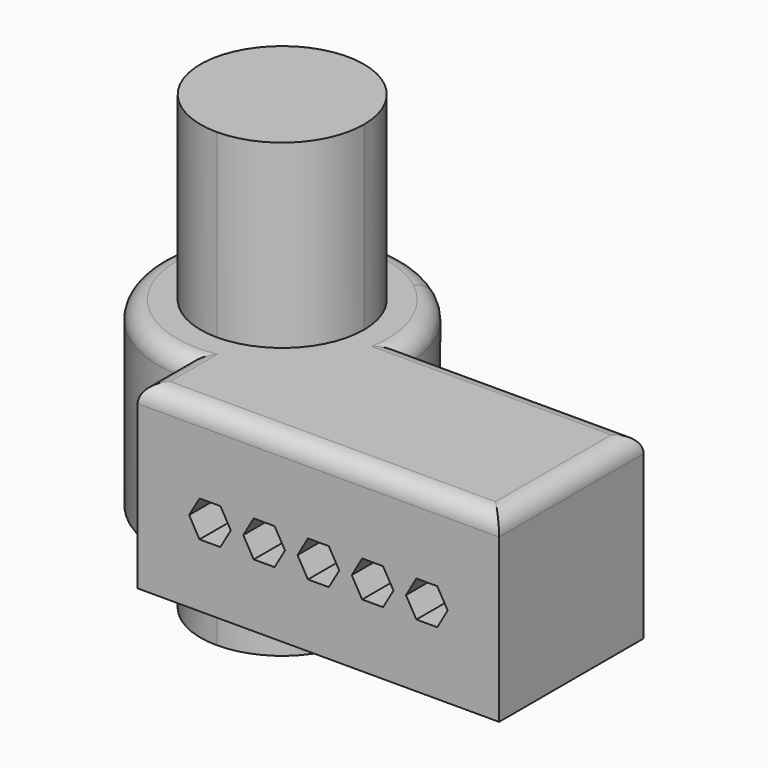
from build123d import *

# Parameters (mm, degrees)
F1_DEPTH      = 50
F2_DEPTH      = 100
F2_DEPTH_BACK = 25
F3_R          = 5
F5_DEPTH      = 84.1452189972


with BuildPart() as f1:
    # F0 (on Top) → F1 (new body)
    with BuildSketch(Plane.XY):
        with BuildLine():
            ThreePointArc((-42.5412729383, -0.0076430535), (-58.519124099, 38.5663019163), (-19.9451791292, 22.5884507556))
            Line((-19.9451791292, 22.5884507556), (-8.397054041, 22.5884507556))
            ThreePointArc((-8.397054041, 22.5884507556), (-11.8913995751, 37.6354752761), (-21.6592081763, 49.6026517502))
            ThreePointArc((-21.6592081763, 49.6026517502), (-74.853859311, 33.621330978), (-42.5412729383, -11.5557681416))
            Line((-42.5412729383, -11.5557681416), (-42.5412729383, -0.0076430535))
        make_face()
        with BuildLine():
            Line((57.4587270617, 22.5884507556), (-8.397054041, 22.5884507556))
            ThreePointArc((-8.397054041, 22.5884507556), (-18.3976642177, -1.555157965), (-42.5412729383, -11.5557681416))
            Line((-42.5412729383, -11.5557681416), (-42.5412729383, -27.4115492444))
            Line((-42.5412729383, -27.4115492444), (57.4587270617, -27.4115492444))
            Line((57.4587270617, -27.4115492444), (57.4587270617, 22.5884507556))
        make_face()
        with BuildLine():
            Line((-8.397054041, 22.5884507556), (-19.9451791292, 22.5884507556))
            ThreePointArc((-19.9451791292, 22.5884507556), (-26.5634217775, 6.6105995948), (-42.5412729383, -0.0076430535))
            Line((-42.5412729383, -0.0076430535), (-42.5412729383, -11.5557681416))
            ThreePointArc((-42.5412729383, -11.5557681416), (-18.3976642177, -1.555157965), (-8.397054041, 22.5884507556))
        make_face()
    extrude(amount=F1_DEPTH)

    # F3
    f3_edges = [f1.edges().sort_by_distance(p)[0] for p in [
        (7.458727, -27.411549, 50),
        (-42.541273, -19.483659, 50),
        (-66.684882, 46.732059, 50),
        (24.530837, 22.588451, 50),
        (57.458727, -2.411549, 50),
    ]]
    fillet(f3_edges, radius=F3_R)

    # F4 (on face) → F5 (cut, through all)
    with BuildSketch(Plane.XZ.offset(27.4115492444)):
        Polygon((-19.6545215923, 17.5), (-16.7677702464, 22.5), (-19.6545215923, 27.5), (-25.4280242842, 27.5), (-28.3147756301, 22.5), (-25.4280242842, 17.5), align=None)
        Polygon((-4.6545215923, 27.5), (-10.4280242842, 27.5), (-13.3147756301, 22.5), (-10.4280242842, 17.5), (-4.6545215923, 17.5), (-1.7677702464, 22.5), align=None)
        Polygon((10.3454784077, 27.5), (4.5719757158, 27.5), (1.6852243699, 22.5), (4.5719757158, 17.5), (10.3454784077, 17.5), (13.2322297536, 22.5), align=None)
        Polygon((25.3454784077, 27.5), (19.5719757158, 27.5), (16.6852243699, 22.5), (19.5719757158, 17.5), (25.3454784077, 17.5), (28.2322297536, 22.5), align=None)
        Polygon((40.3454784077, 27.5), (34.5719757158, 27.5), (31.6852243699, 22.5), (34.5719757158, 17.5), (40.3454784077, 17.5), (43.2322297536, 22.5), align=None)
    extrude(amount=-F5_DEPTH, mode=Mode.SUBTRACT)


with BuildPart() as f2:
    # F0 (on Top) → F2 (new body, two sides)
    with BuildSketch(Plane.XY) as f2_sk:
        with BuildLine():
            Line((-42.5412729383, -0.0076430535), (-42.5412729383, 22.5884507556))
            Line((-42.5412729383, 22.5884507556), (-19.9451791292, 22.5884507556))
            ThreePointArc((-19.9451791292, 22.5884507556), (-58.519124099, 38.5663019163), (-42.5412729383, -0.0076430535))
        make_face()
        with BuildLine():
            Line((-19.9451791292, 22.5884507556), (-42.5412729383, 22.5884507556))
            Line((-42.5412729383, 22.5884507556), (-42.5412729383, -0.0076430535))
            ThreePointArc((-42.5412729383, -0.0076430535), (-26.5634217775, 6.6105995948), (-19.9451791292, 22.5884507556))
        make_face()
    extrude(amount=F2_DEPTH)
    extrude(f2_sk.sketch, amount=-F2_DEPTH_BACK)


solid = Compound([f1.part, f2.part])
